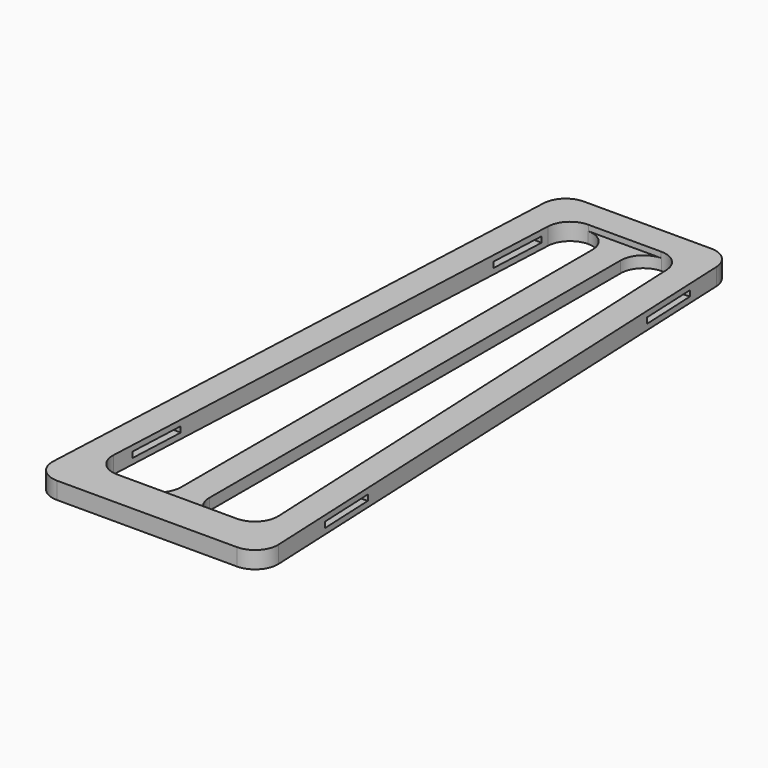
from build123d import *

# Parameters (mm, degrees)
F1_DEPTH = 3.81
F0_W     = 6.35
F0_H     = 124.968
F2_DEPTH = 2.54
F3_W     = 12.7
F3_H     = 1.27
F4_DEPTH = 6.35
F5_W     = 12.7
F5_H     = 1.27
F6_DEPTH = 6.35
F7_F1_R  = 5.08
F7_F2_R  = 5.08
F7_F3_R  = 5.08
F7_F4_R  = 5.08
F7_F5_R  = 5.08
F7_F6_R  = 5.08
F7_F7_R  = 5.08
F7_F8_R  = 5.08
F7_F9_R  = 5.08
F7_F10_R = 5.08
F7_F11_R = 5.08
F7_F12_R = 5.08


with BuildPart() as f1:
    # F0 (on Top) → F1 (new body)
    with BuildSketch(Plane.XY):
        Polygon((6.35, 139.7), (0, 0), (50.8, 0), (44.45, 139.7), align=None)
        Polygon((38.3820798312, 133.35), (44.0624434675, 8.382), (28.575, 8.382), (22.225, 8.382), (6.7375565325, 8.382), (12.4179201688, 133.35), (22.225, 133.35), (28.575, 133.35), align=None, mode=Mode.SUBTRACT)
    extrude(amount=F1_DEPTH)

    # F0 (on Top) → F2 (join)
    with BuildSketch(Plane.XY):
        with Locations((25.4, 70.866)):
            Rectangle(F0_W, F0_H)
    extrude(amount=F2_DEPTH)

    # F3 (on face) → F4 (cut)
    with BuildSketch(Plane(origin=(0, 0, 0), x_dir=(-0.0454076609, -0.9989685402, 0), z_dir=(-0.9989685402, 0.0454076609, 0))):
        with Locations((-120.7942437142, 1.905)):
            Rectangle(F3_W, F3_H)
        with Locations((-25.4, 1.905)):
            Rectangle(F3_W, F3_H)
    extrude(amount=-F4_DEPTH, mode=Mode.SUBTRACT)

    # F5 (on face) → F6 (cut)
    with BuildSketch(Plane(origin=(50.695257732, 2.3043298969, 0), x_dir=(-0.0454076609, 0.9989685402, 0), z_dir=(0.9989685402, 0.0454076609, 0))):
        with Locations((23.0932908253, 1.905)):
            Rectangle(F5_W, F5_H)
        with Locations((118.4875345395, 1.905)):
            Rectangle(F5_W, F5_H)
    extrude(amount=-F6_DEPTH, mode=Mode.SUBTRACT)

    # F7: fillet of radius 5.08 on 12 edges, made by hand

    # F7_f1
    f7_f1_edges = [f1.edges().sort_by_distance(p)[0] for p in [
        (28.575, 8.382, 1.27),
    ]]
    fillet(f7_f1_edges, radius=F7_F1_R)

    # F7_f2
    f7_f2_edges = [f1.edges().sort_by_distance(p)[0] for p in [
        (22.225, 8.382, 1.27),
    ]]
    fillet(f7_f2_edges, radius=F7_F2_R)

    # F7_f3
    f7_f3_edges = [f1.edges().sort_by_distance(p)[0] for p in [
        (28.575, 133.35, 1.27),
    ]]
    fillet(f7_f3_edges, radius=F7_F3_R)

    # F7_f4
    f7_f4_edges = [f1.edges().sort_by_distance(p)[0] for p in [
        (22.225, 133.35, 1.27),
    ]]
    fillet(f7_f4_edges, radius=F7_F4_R)

    # F7_f5
    f7_f5_edges = [f1.edges().sort_by_distance(p)[0] for p in [
        (6.35, 139.7, 1.905),
    ]]
    fillet(f7_f5_edges, radius=F7_F5_R)

    # F7_f6
    f7_f6_edges = [f1.edges().sort_by_distance(p)[0] for p in [
        (0, 0, 1.905),
    ]]
    fillet(f7_f6_edges, radius=F7_F6_R)

    # F7_f7
    f7_f7_edges = [f1.edges().sort_by_distance(p)[0] for p in [
        (44.45, 139.7, 1.905),
    ]]
    fillet(f7_f7_edges, radius=F7_F7_R)

    # F7_f8
    f7_f8_edges = [f1.edges().sort_by_distance(p)[0] for p in [
        (50.8, 0, 1.905),
    ]]
    fillet(f7_f8_edges, radius=F7_F8_R)

    # F7_f9
    f7_f9_edges = [f1.edges().sort_by_distance(p)[0] for p in [
        (38.3820798312, 133.35, 1.905),
    ]]
    fillet(f7_f9_edges, radius=F7_F9_R)

    # F7_f10
    f7_f10_edges = [f1.edges().sort_by_distance(p)[0] for p in [
        (44.0624434675, 8.382, 1.905),
    ]]
    fillet(f7_f10_edges, radius=F7_F10_R)

    # F7_f11
    f7_f11_edges = [f1.edges().sort_by_distance(p)[0] for p in [
        (6.7375565325, 8.382, 1.905),
    ]]
    fillet(f7_f11_edges, radius=F7_F11_R)

    # F7_f12
    f7_f12_edges = [f1.edges().sort_by_distance(p)[0] for p in [
        (12.4179201688, 133.35, 1.905),
    ]]
    fillet(f7_f12_edges, radius=F7_F12_R)


solid = f1.part
